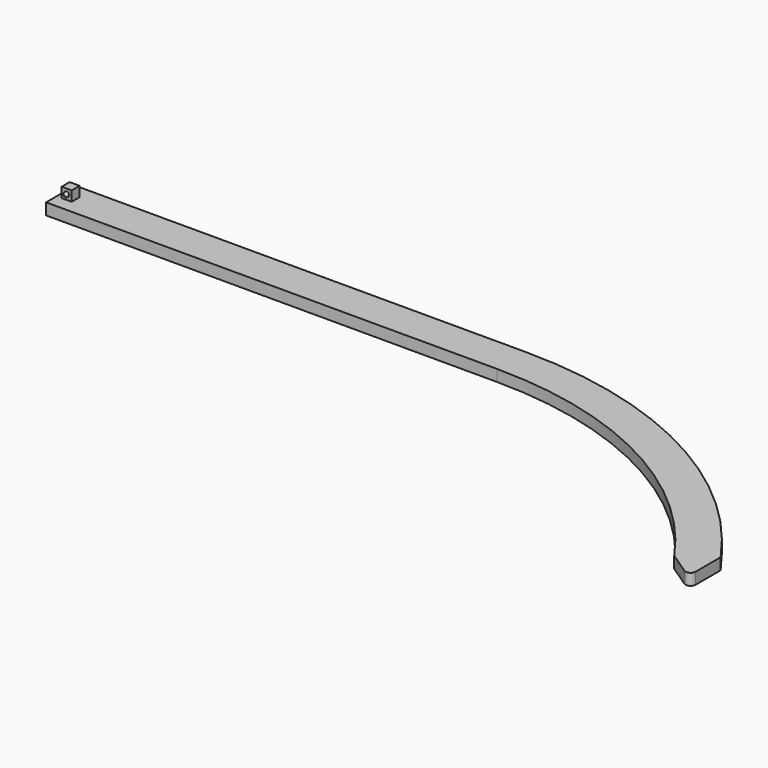
from build123d import *

# Parameters (mm, degrees)
F1_DEPTH = 2.3
F3_DEPTH = 2


with BuildPart() as f1:
    # F0 (on Top) → F1 (new body)
    with BuildSketch(Plane.XY):
        Polygon((45, 3.625), (-45, 3.625), (-45, 0), (-45, -3.625), (45, -3.625), align=None)
        Polygon((-44, -1), (-44, 0), (-44, 1), (-42, 1), (-42, -1), align=None, mode=Mode.SUBTRACT)
        with BuildLine():
            ThreePointArc((111.9139716029, -31.496938318), (82.7856789898, -5.6889854515), (45, 3.625))
            Line((45, 3.625), (45, -3.625))
            ThreePointArc((45, -3.625), (79.4162271285, -12.1084320129), (105.947070592, -35.615019464))
            Line((105.947070592, -35.615019464), (110.3610228539, -38.574432601))
            ThreePointArc((110.3610228539, -38.574432601), (111.3860089549, -38.6260052928), (111.9139716029, -37.7459418336))
            Line((111.9139716029, -37.7459418336), (111.9139716029, -31.496938318))
        make_face()
        Polygon((-44, 1), (-44, 0), (-44, -1), (-42, -1), (-42, 1), align=None)
    extrude(amount=F1_DEPTH)

    # F2 (on face) → F3 (join)
    with BuildSketch(Plane.XY.offset(2.3)):
        Polygon((-44, 1), (-44, 0), (-44, -1), (-42, -1), (-42, 1), align=None)
    extrude(amount=F3_DEPTH)

    # F6 (on face) → F7 (revolve)
    with BuildSketch(Plane.XZ.offset(1)):
        with BuildLine():
            ThreePointArc((-42.5, 3.3), (-42.6464466094, 3.6535533906), (-43, 3.8))
            Line((-43, 3.8), (-43, 3.3))
            Line((-43, 3.3), (-42.5, 3.3))
        make_face()
        with BuildLine():
            Line((-42.5, 3.3), (-43, 3.3))
            Line((-43, 3.3), (-43, 2.8))
            ThreePointArc((-43, 2.8), (-42.6464466094, 2.9464466094), (-42.5, 3.3))
        make_face()
    revolve(axis=Axis((-43, -1, 3.3), (0, 0, -1)))


with BuildPart() as f5:
    # F4 (on face) → F5 (revolve)
    with BuildSketch(Plane(origin=(0, 1, 0), x_dir=(-1, 0, 0), z_dir=(0, 1, 0))):
        with BuildLine():
            Line((43, 3.3), (43.5, 3.3))
            ThreePointArc((43.5, 3.3), (43.3535533906, 3.6535533906), (43, 3.8))
            Line((43, 3.8), (43, 3.3))
        make_face()
        with BuildLine():
            ThreePointArc((43, 2.8), (43.3535533906, 2.9464466094), (43.5, 3.3))
            Line((43.5, 3.3), (43, 3.3))
            Line((43, 3.3), (43, 2.8))
        make_face()
    revolve(axis=Axis((-43, 1, 3.3), (0, 0, -1)))


solid = Compound([f1.part, f5.part])
